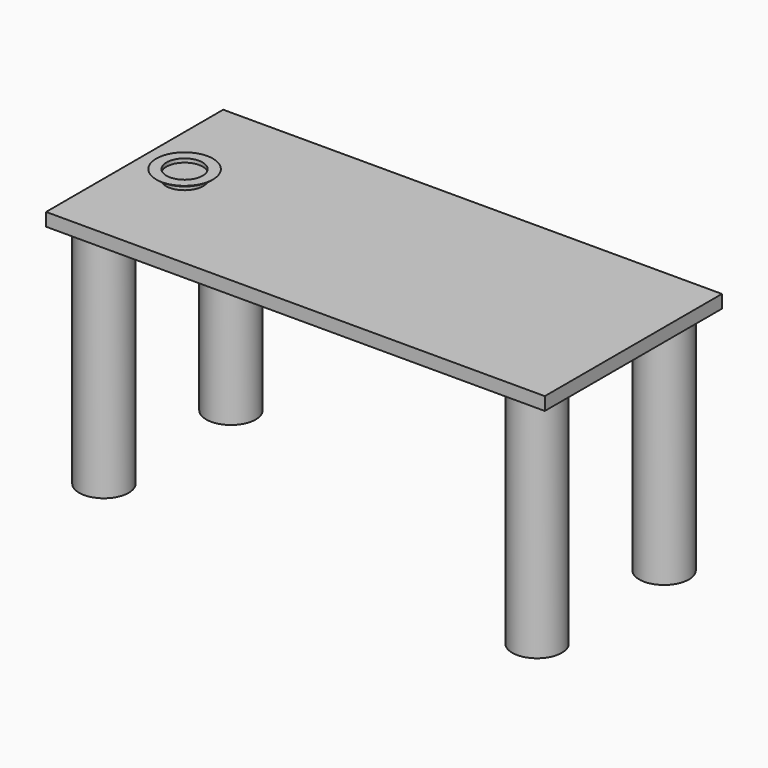
from build123d import *

# Parameters (mm, degrees)
F0_W      = 133.715108037
F0_H      = 59.3623146415
F1_DEPTH  = 3.5
F2_R      = 6.6440898667
F3_DEPTH  = 61.2
F4_R      = 4.997826556
F5_DEPTH  = 1.4
F6_R      = 7.6010927322
F7_DEPTH  = 1
F9_R      = 4.8490813771
F10_DEPTH = 1


# Not quite as in the source:
# - a fillet or chamfer that OpenCascade refuses, or shapes differently, is made with other operations: its cross-section is extruded or revolved along the edge and cut away or added


with BuildPart() as f1:
    # F0 (on Top) → F1 (new body)
    with BuildSketch(Plane.XY):
        Rectangle(F0_W, F0_H)
    extrude(amount=F1_DEPTH)

    # F2 (on face) → F3 (join)
    with BuildSketch(Plane(origin=(0, 0, 0), x_dir=(1, 0, 0), z_dir=(0, 0, -1))):
        with Locations((-58.0631382763, 21.2864857167)):
            Circle(F2_R)
        with Locations((-58.0631382763, -21.2864857167)):
            Circle(F2_R)
        with Locations((58.0631382763, 21.2864857167)):
            Circle(F2_R)
        with Locations((58.0631382763, -21.2864857167)):
            Circle(F2_R)
    extrude(amount=F3_DEPTH)

    # F4 (on face) → F5 (join)
    with BuildSketch(Plane.XY.offset(3.5)):
        with Locations((-53.4660555422, 0)):
            Circle(F4_R)
    extrude(amount=F5_DEPTH)

    # F6 (on face) → F7 (join)
    with BuildSketch(Plane.XY.offset(4.9)):
        with Locations((-53.4660555422, 0)):
            Circle(F6_R)
    extrude(amount=F7_DEPTH)

    # F8: fillet of radius 3.6213203436 on 1 edges, made by hand

    # F8_s1 → F8_t2 (revolve, cut)
    with BuildSketch(Plane.XZ):
        with BuildLine():
            ThreePointArc((-45.86496281, 5.9), (-47.0178827806, 5.1592821435), (-48.3634905139, 4.9))
            Line((-48.3634905139, 4.9), (-45.86496281, 4.9))
            Line((-45.86496281, 4.9), (-45.86496281, 5.9))
        make_face()
    revolve(axis=Axis((-53.4660555422, 0, 4.9), (0, 0, 1)), mode=Mode.SUBTRACT)

    # F9 (on face) → F10 (cut)
    with BuildSketch(Plane.XY.offset(5.9)):
        with Locations((-53.4660555422, 0)):
            Circle(F9_R)
    extrude(amount=-F10_DEPTH, mode=Mode.SUBTRACT)


solid = f1.part
